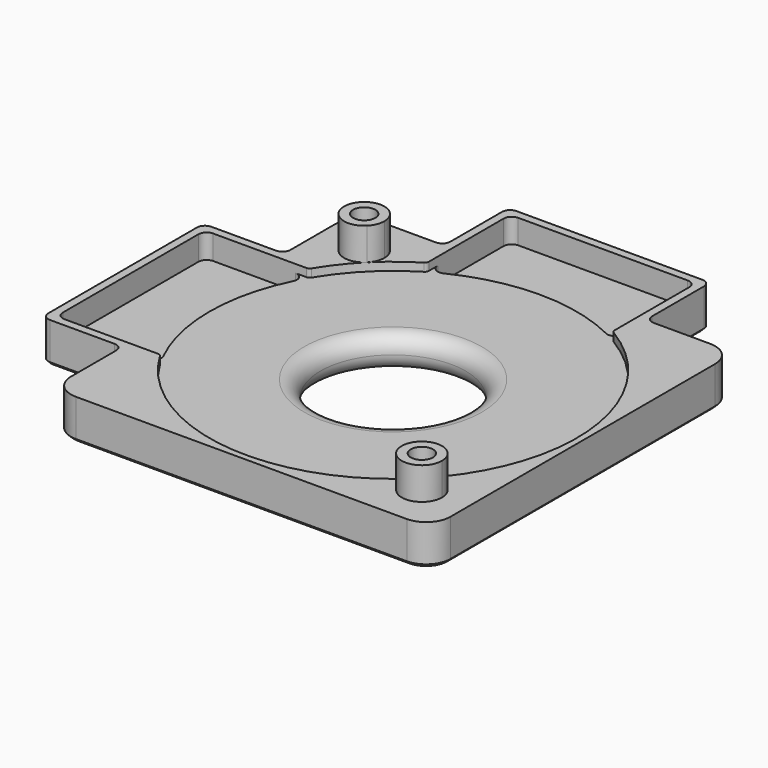
from build123d import *

# Parameters (mm, degrees)
F1_DEPTH        = 5
F2_R            = 22.75
F3_DEPTH        = 1
F5_DEPTH        = 4
F6_DEPTH        = 3
F7_R            = 9
F8_DEPTH        = 4.001
F9_R            = 3
F10_R           = 1
F11_R           = 0.5
F13_D           = 2.75
F13_CBORE_D     = 4.6
F13_CBORE_DEPTH = 2
F14_R           = 1.99999
F15_SIZE        = 0.4
F16_ANGLE       = 180


# Not quite as in the source:
# - a fillet or chamfer is up to 0.001 mm smaller than in the source, because OpenCascade refuses the exact size


with BuildPart() as f1:
    # F0 (on Top) → F1 (new body)
    with BuildSketch(Plane.XY):
        Polygon((23.5, -23.5), (23.5, 23.5), (-23.5, 23.5), (-23.5, 12.5), (-33.5, 12.5), (-33.5, -12.5), (-23.5, -12.5), (-23.5, -23.5), (-12.5, -23.5), (-12.5, -33.5), (12.5, -33.5), (12.5, -23.5), align=None)
    extrude(amount=F1_DEPTH)

    # F2 (on face) → F3 (cut)
    with BuildSketch(Plane(origin=(0, 0, 0), x_dir=(1, 0, 0), z_dir=(0, 0, -1))):
        Circle(F2_R)
    extrude(amount=-F3_DEPTH, mode=Mode.SUBTRACT)

    # F4 (on face) → F5 (join)
    with BuildSketch(Plane.XY):
        with BuildLine():
            ThreePointArc((-16.086679292, -16.086679252), (-20.153889553, -18.8043023144), (-15.3562879116, -17.85))
            ThreePointArc((-15.3562879116, -17.85), (-15.546110447, -16.8956976856), (-16.086679292, -16.086679252))
        make_face()
        with BuildLine():
            ThreePointArc((20.3437120884, 17.85), (16.8956976987, 20.1538895584), (16.086679272, 16.086679272))
            ThreePointArc((16.086679272, 16.086679272), (18.8043023013, 15.5461104416), (20.3437120884, 17.85))
        make_face()
    extrude(amount=-F5_DEPTH)

    # F4 (on face) → F6 (cut)
    with BuildSketch(Plane.XY):
        with BuildLine():
            ThreePointArc((11.5, -19.6293784925), (0, -22.75), (-11.5, -19.6293784925))
            Line((-11.5, -19.6293784925), (-11.5, -32.5))
            Line((-11.5, -32.5), (11.5, -32.5))
            Line((11.5, -32.5), (11.5, -19.6293784925))
        make_face()
        with BuildLine():
            Line((-32.5, -11.5), (-19.6293784925, -11.5))
            ThreePointArc((-19.6293784925, -11.5), (-22.75, 0), (-19.6293784925, 11.5))
            Line((-19.6293784925, 11.5), (-32.5, 11.5))
            Line((-32.5, 11.5), (-32.5, -11.5))
        make_face()
    extrude(amount=F6_DEPTH, mode=Mode.SUBTRACT)

    # F7 (on face) → F8 (cut, through all)
    with BuildSketch(Plane(origin=(0, 0, 1), x_dir=(1, 0, 0), z_dir=(0, 0, -1))):
        Circle(F7_R)
    extrude(amount=-F8_DEPTH, mode=Mode.SUBTRACT)

    # F9
    f9_edges = [f1.edges().sort_by_distance(p)[0] for p in [
        (-23.5, 23.5, 2.5),
        (23.5, 23.5, 2.5),
        (23.5, -23.5, 2.5),
        (-23.5, -23.5, 2.5),
    ]]
    fillet(f9_edges, radius=F9_R)

    # F10
    f10_edges = [f1.edges().sort_by_distance(p)[0] for p in [
        (-32.5, -11.5, 1.5),
        (-33.5, 12.5, 2.5),
        (-32.5, 11.5, 1.5),
        (-33.5, -12.5, 2.5),
        (-12.5, -33.5, 2.5),
        (12.5, -33.5, 2.5),
        (-11.5, -32.5, 1.5),
        (11.5, -32.5, 1.5),
        (-23.5, -12.5, 2.5),
        (-23.5, 12.5, 2.5),
        (-12.5, -23.5, 2.5),
        (12.5, -23.5, 2.5),
        (-19.629378, -11.5, 2),
        (-19.629378, 11.5, 2),
        (11.5, -19.629378, 2),
        (-11.5, -19.629378, 2),
    ]]
    fillet(f10_edges, radius=F10_R)

    # F11
    f11_edges = [f1.edges().sort_by_distance(p)[0] for p in [
        (-19.629378, -11.5, 0.5),
        (-11.5, -19.629378, 0.5),
        (11.5, -19.629378, 0.5),
        (-19.629378, 11.5, 0.5),
    ]]
    fillet(f11_edges, radius=F11_R)

    # F13 (through all)
    with Locations(Plane.XY.offset(5)):
        with Locations((-17.85, -17.85), (17.85, 17.85)):
            CounterBoreHole(F13_D / 2, F13_CBORE_D / 2, F13_CBORE_DEPTH)

    # F14 (radius 2 in the source; OpenCascade refuses exactly that, so slightly less here)
    f14_edges = [f1.edges().sort_by_distance(p)[0] for p in [
        (-9, 0, 5),
        (-9, 0, 1),
    ]]
    fillet(f14_edges, radius=F14_R)

    # F15
    f15_edges = [f1.edges().sort_by_distance(p)[0] for p in [
        (-33.5, 0, 5),
    ]]
    chamfer(f15_edges, length=F15_SIZE)


with BuildPart() as f1_1:
    # F16: moved
    add(f1.part.rotate(Axis((0, -33.5, 0), (-1, 0, 0)), F16_ANGLE))


with BuildPart() as f1_2:
    # F17: moved
    add(f1_1.part.moved(Location((0, 50, 0))))


solid = f1_2.part
